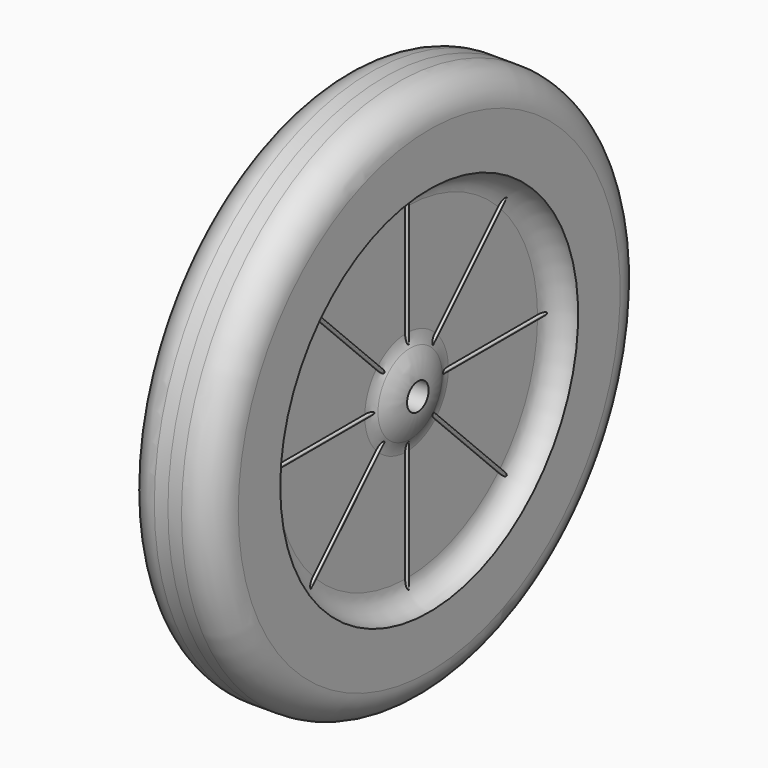
from build123d import *

# Parameters (mm, degrees)
F2_R          = 6.35
F4_DEPTH      = 0.635
F5_R          = 0.5079
F7_R          = 8.89
F8_R          = 3.81
F9_DEPTH      = 25.4
F9_DEPTH_BACK = 25.4


# Not quite as in the source:
# - a fillet or chamfer is up to 0.001 mm smaller than in the source, because OpenCascade refuses the exact size
# - a feature names something its author has since deleted; it is built from what else it names


with BuildPart() as f1:
    # F0 (on Top) → F1 (revolve)
    with BuildSketch(Plane.XY):
        with BuildLine():
            Line((-6.3056110429, -12.7449716337), (-6.3056110429, -52.5464490056))
            Line((-6.3056110429, -52.5464490056), (-12.7304934542, -52.5464490056))
            Line((-12.7304934542, -52.5464490056), (-12.7304934542, -76.2437978662))
            Line((-12.7304934542, -76.2437978662), (12.7304934542, -76.2620939388))
            Line((12.7304934542, -76.2620939388), (12.7304934542, -63.5529825109))
            Line((12.7304934542, -63.5529825109), (12.7304934542, -52.5464490056))
            Line((12.7304934542, -52.5464490056), (6.3486411236, -52.5464490056))
            Line((6.3486411236, -52.5464490056), (6.3486411236, -12.6927555603))
            ThreePointArc((6.3486411236, -12.6927555603), (8.7070293588, -8.5267945168), (9.525, -3.81))
            ThreePointArc((9.525, -3.81), (11.8172948862, -2.4923290719), (12.7, 0))
            Line((12.7, 0), (-9.525, 0))
            Line((-9.525, 0), (-9.525, -3.81))
            ThreePointArc((-9.525, -3.81), (-8.6955997963, -8.5586362082), (-6.3056110429, -12.7449716337))
        make_face()
        with BuildLine():
            ThreePointArc((-12.7, 0), (-11.8172948862, -2.4923290719), (-9.525, -3.81))
            Line((-9.525, -3.81), (-9.525, 0))
            Line((-9.525, 0), (-12.7, 0))
        make_face()
    revolve(axis=Axis((0, 0, 0), (1, 0, 0)))

    # F2
    f2_edges = [f1.edges().sort_by_distance(p)[0] for p in [
        (6.348641, 12.692756, 0),
        (6.348641, 52.546449, 0),
    ]]
    fillet(f2_edges, radius=F2_R)

    # F3 (on face) → F4 (join)
    with BuildSketch(Plane(origin=(-6.3056110429, 0, 0), x_dir=(0, -1, 0), z_dir=(-1, 0, 0))):
        Polygon((-1.2264204897, -0.508), (-0.7184204897, 0), (-46.1964490056, 0), (-46.193655806, -0.508), align=None)
        Polygon((-1.2264204897, 0.508), (-0.7184204897, 0), (-0.508, 0.2104204897), (-0.508, 0.508), align=None)
        Polygon((-0.508, -0.2104204897), (-0.7184204897, 0), (-1.2264204897, -0.508), (-0.508, -0.508), align=None)
        Polygon((-46.1964490056, 0), (-0.7184204897, 0), (-1.2264204897, 0.508), (-46.193655806, 0.508), align=None)
        Polygon((-0.508, 0.508), (-0.2104204897, 0.508), (0, 0.7184204897), (-0.508, 1.2264204897), align=None)
        Polygon((0, 0.7184204897), (0.2104204897, 0.508), (0.508, 0.508), (0.508, 1.2264204897), align=None)
        Polygon((0, -0.7184204897), (-0.2104204897, -0.508), (-0.508, -0.508), (-0.508, -1.2264204897), align=None)
        Polygon((0.508, -0.508), (0.2104204897, -0.508), (0, -0.7184204897), (0.508, -1.2264204897), align=None)
        Polygon((0.7184204897, 0), (0.508, -0.2104204897), (0.508, -0.508), (1.2264204897, -0.508), align=None)
        Polygon((0.508, 0.508), (0.508, 0.2104204897), (0.7184204897, 0), (1.2264204897, 0.508), align=None)
        Polygon((-46.193655806, -0.508), (-46.1964490056, 0), (-46.193655806, 0.508), (-49.4300462306, 0.508), (-49.4300462306, -0.508), align=None)
        Polygon((-0.508, -0.508), (-1.2264204897, -0.508), (-35.3115311288, -34.5931106391), (-34.5931106391, -35.3115311288), (-32.3046370234, -33.0230575131), (-0.508, -1.2264204897), align=None)
        Polygon((-33.0230575131, 32.3046370234), (-1.2264204897, 0.508), (-0.508, 0.508), (-0.508, 1.2264204897), (-34.5931106391, 35.3115311288), (-35.3115311288, 34.5931106391), align=None)
        Polygon((-0.508, 1.2264204897), (0, 0.7184204897), (0.508, 1.2264204897), (0.508, 49.4300462306), (-0.508, 49.4300462306), (-0.508, 46.193655806), align=None)
        Polygon((0.508, 1.2264204897), (0.508, 0.508), (1.2264204897, 0.508), (35.3115311288, 34.5931106391), (34.5931106391, 35.3115311288), (32.3046370234, 33.0230575131), align=None)
        Polygon((0.508, -1.2264204897), (0, -0.7184204897), (-0.508, -1.2264204897), (-0.508, -49.4300462306), (0.508, -49.4300462306), (0.508, -46.193655806), align=None)
        Polygon((1.2264204897, -0.508), (0.508, -0.508), (0.508, -1.2264204897), (34.5931106391, -35.3115311288), (35.3115311288, -34.5931106391), (33.0230575131, -32.3046370234), align=None)
        Polygon((1.2264204897, 0.508), (0.7184204897, 0), (1.2264204897, -0.508), (49.4300462306, -0.508), (49.4300462306, 0.508), (46.193655806, 0.508), align=None)
    extrude(amount=F4_DEPTH)

    # F5 (radius 0.508 in the source; OpenCascade refuses exactly that, so slightly less here)
    f5_edges = [f1.edges().sort_by_distance(p)[0] for p in [
        (-6.940611, 30.668254, -0.508),
        (-6.940611, 0.508, 30.668254),
        (-6.940611, -21.32652, 22.044941),
        (-6.940611, 22.044941, 21.32652),
        (-6.940611, -30.668254, 0.508),
        (-6.940611, -22.044941, -21.32652),
        (-6.940611, -0.508, -30.668254),
        (-6.940611, 21.32652, -22.044941),
        (-6.940611, -30.668254, -0.508),
        (-6.940611, -22.044941, 21.32652),
        (-6.940611, -0.508, 30.668254),
        (-6.940611, 21.32652, 22.044941),
        (-6.940611, 30.668254, 0.508),
        (-6.940611, 22.044941, -21.32652),
        (-6.940611, 0.508, -30.668254),
        (-6.940611, -21.32652, -22.044941),
    ]]
    fillet(f5_edges, radius=F5_R)

    # F6: F1 across plane


with BuildPart() as f1_1:
    add(f1.part)
    add(f1.part.mirror(Plane.YZ))

    # F7
    f7_edges = [f1_1.edges().sort_by_distance(p)[0] for p in [
        (12.730493, 76.262094, 0),
        (-12.730493, 76.262094, 0),
    ]]
    fillet(f7_edges, radius=F7_R)

    # F8 (on Right) → F9 (cut, two sides)
    with BuildSketch(Plane.YZ) as f9_sk:
        Circle(F8_R)
    extrude(amount=-F9_DEPTH, mode=Mode.SUBTRACT)
    extrude(f9_sk.sketch, amount=F9_DEPTH_BACK, mode=Mode.SUBTRACT)


solid = f1_1.part
